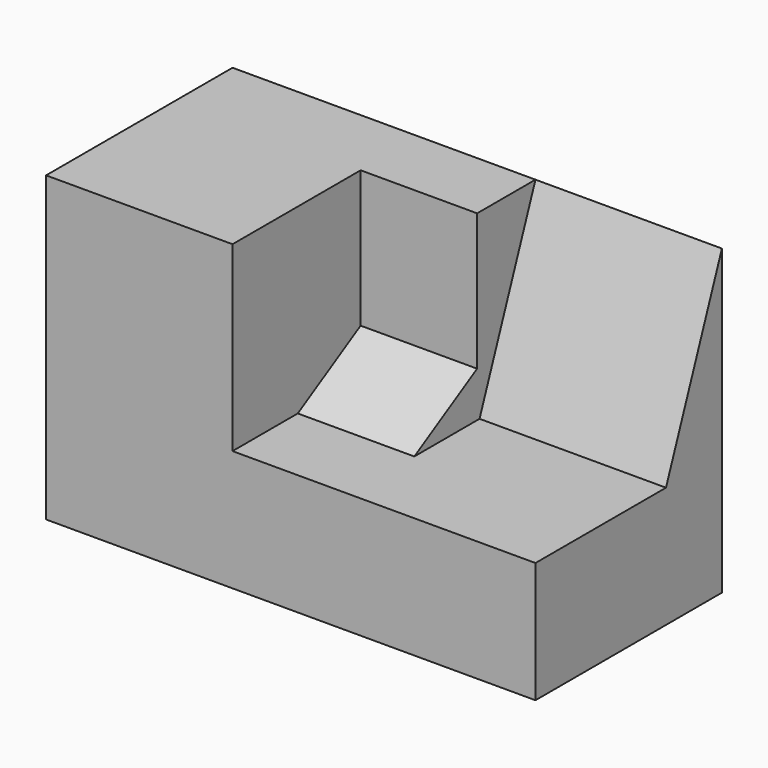
from build123d import *

# Parameters (mm, degrees)
F0_W     = 105
F0_H     = 65
F1_DEPTH = 50
F3_DEPTH = 40
F5_DEPTH = 25
F6_DEPTH = 25
F7_DEPTH = 25


# Not quite as in the source:
# - a feature names something its author has since deleted; it is built from what else it names


with BuildPart() as f1:
    # F0 (on Front) → F1 (new body)
    with BuildSketch(Plane.XZ):
        Rectangle(F0_W, F0_H)
    extrude(amount=-F1_DEPTH)

    # F2 (on face) → F3 (cut)
    with BuildSketch(Plane.YZ.offset(52.5)):
        Polygon((0, 32.5), (0, -6.5763359704), (35, -6.5763359704), (50, 32.5), align=None)
    extrude(amount=-F3_DEPTH, mode=Mode.SUBTRACT)

    # F4 (on face) → F5 (join)
    with BuildSketch(Plane.YZ.offset(12.5)):
        Polygon((34.35340128, 3.1539797953), (34.35340128, 32.5), (0, 32.5), (0, -6.5763359704), (17.5, -6.5763359704), align=None)
    extrude(amount=-F5_DEPTH)

    # F4 (on face) → F6 (join)
    with BuildSketch(Plane.YZ.offset(12.5)):
        Polygon((34.35340128, 3.1539797953), (34.35340128, 32.5), (0, 32.5), (0, -6.5763359704), (17.5, -6.5763359704), align=None)
    extrude(amount=-F6_DEPTH)

    # F4 (on face) → F7 (cut)
    with BuildSketch(Plane.YZ.offset(12.5)):
        Polygon((34.35340128, 3.1539797953), (34.35340128, 32.5), (0, 32.5), (0, -6.5763359704), (17.5, -6.5763359704), align=None)
    extrude(amount=-F7_DEPTH, mode=Mode.SUBTRACT)


solid = f1.part
